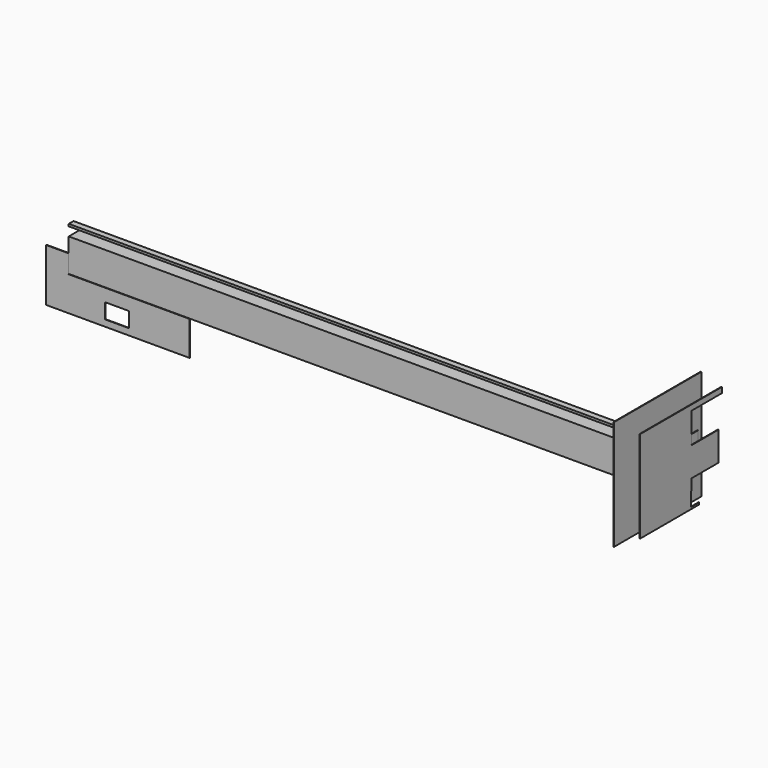
from build123d import *

# Parameters (mm, degrees)
F0_W      = 1666.3101315498
F0_H      = 1440.3567910194
F0_W_2    = 321.9513893127
F0_H_2    = 173.8705039024
F1_DEPTH  = 25.4
F2_W      = 601.3025641441
F2_H      = 270.2689170837
F2_W_2    = 546.2159514427
F2_H_2    = 393.4317827225
F2_W_3    = 484.9420785904
F2_H_3    = 512.361317873
F2_W_4    = 315.6808614731
F2_H_4    = 497.0915317535
F2_W_5    = 263.4772062302
F2_H_5    = 414.9414896965
F3_DEPTH  = 25.4
F4_W      = 1832.0484161377
F4_H      = 3807.0937395096
F5_DEPTH  = 25.4
F6_W      = 670.0121164322
F6_H      = 1531.9002270699
F6_W_2    = 276.8320441246
F6_H_2    = 106.2819361687
F7_DEPTH  = 28066.4691925049
F8_W      = 5071.1117982864
F8_H      = 5097.4462032318
F9_DEPTH  = 25.4
F10_W     = 1443.1173034668
F10_H     = 1491.5601015091
F10_W_2   = 1109.7354888916
F10_H_2   = 703.5193443298
F10_W_3   = 2133.3904266357
F10_H_3   = 1594.1830873489
F11_DEPTH = 25.4
F12_W     = 2353.1031608582
F12_H     = 645.3219652176
F12_H_2   = 89.3001556396
F12_W_2   = 1552.1093606949
F12_H_3   = 1351.4214754105
F12_W_3   = 466.8933153152
F13_DEPTH = 25.4


with BuildPart() as f1:
    # F0 (on Right) → F1 (new body)
    with BuildSketch(Plane.YZ):
        with Locations((-82.8691422939, -112.1042668819)):
            Rectangle(F0_W, F0_H)
        with Locations((160.9756946564, 86.9352519512)):
            Rectangle(F0_W_2, F0_H_2, mode=Mode.SUBTRACT)
    extrude(amount=F1_DEPTH)

    # F2 (on face) → F3 (join)
    with BuildSketch(Plane.YZ.offset(25.4)):
        Polygon((601.3025641441, -1092.7692651749), (901.9212722778, -1092.7692651749), (901.9212722778, -524.1619944572), (901.9212722778, 428.5740554333), (901.9212722778, 856.0312390327), (-642.5161361694, 856.0312390327), (-1059.429526329, 856.0312390327), (-1059.429526329, 658.6785316467), (-1059.429526329, 243.7370419502), (-1059.429526329, -191.7653083801), (-1059.429526329, -688.8568401337), (-1059.429526329, -1092.7692651749), (-1031.0319662094, -1092.7692651749), (-484.8160147667, -1092.7692651749), (0, -1092.7692651749), align=None)
        with Locations((300.6512820721, -1227.9037237167)):
            Rectangle(F2_W, F2_H)
        Polygon((901.9212722778, 428.5740554333), (901.9212722778, -524.1619944572), (1412.9276275635, -524.1619944572), (1412.9276275635, 428.5740554333), (927.9855489731, 428.5740554333), align=None)
        Polygon((901.9212722778, 856.0312390327), (901.9212722778, 428.5740554333), (927.9855489731, 428.5740554333), (927.9855489731, 940.9353733063), (-642.5161361694, 940.9353733063), (-642.5161361694, 856.0312390327), align=None)
        with Locations((-757.9239904881, -1289.4851565361)):
            Rectangle(F2_W_2, F2_H_2)
        with Locations((1170.4565882683, 684.7547143698)):
            Rectangle(F2_W_3, F2_H_3)
        Polygon((-1059.429526329, 856.0312390327), (-642.5161361694, 856.0312390327), (-642.5161361694, 940.9353733063), (-642.5161361694, 1006.4268112183), (-1059.429526329, 1006.4268112183), align=None)
        Polygon((-642.5161361694, 940.9353733063), (927.9855489731, 940.9353733063), (927.9855489731, 1309.6973896027), (-642.5161361694, 1309.6973896027), (-642.5161361694, 1006.4268112183), align=None)
        with Locations((-1217.2699570656, -440.3110742569)):
            Rectangle(F2_W_4, F2_H_4)
        with Locations((-1191.1681294441, 451.2077867985)):
            Rectangle(F2_W_5, F2_H_5)
    extrude(amount=F3_DEPTH)

    # F4 (on face) → F5 (join)
    with BuildSketch(Plane(origin=(0, 0, 0), x_dir=(0, -1, 0), z_dir=(-1, 0, 0))):
        with Locations((916.0242080688, 681.5358996391)):
            Rectangle(F4_W, F4_H)
    extrude(amount=F5_DEPTH)

    # F6 (on face) → F7 (join)
    with BuildSketch(Plane(origin=(25.4, 0, 0), x_dir=(0, -1, 0), z_dir=(-1, 0, 0))):
        with Locations((-335.0060582161, -461.9536101818)):
            Rectangle(F6_W, F6_H)
        with Locations((-138.4160220623, 766.5357291698)):
            Rectangle(F6_W_2, F6_H_2)
    extrude(amount=F7_DEPTH)

    # F8 (on face) → F9 (join)
    with BuildSketch(Plane.YZ):
        with Locations((-907.9238772392, 686.8742704391)):
            Rectangle(F8_W, F8_H)
    extrude(amount=F9_DEPTH)

    # F12 (on face) → F13 (join)
    with BuildSketch(Plane.YZ.offset(50.8)):
        Polygon((-1996.6151714325, 2172.7378368378), (-1996.6151714325, 1918.0111885071), (-1375.1103878021, 1918.0111885071), (1005.3068399429, 1918.0111885071), (2760.6105804443, 1918.0111885071), (2760.6105804443, 2172.7378368378), align=None)
        Polygon((-1375.1103878021, 1918.0111885071), (-1996.6151714325, 1918.0111885071), (-1996.6151714325, -2097.6603031158), (-1375.1103878021, -2097.6603031158), (-1375.1103878021, -2008.3601474762), (-1375.1103878021, -1363.0381822586), align=None)
        Polygon((1005.3068399429, 1918.0111885071), (-1375.1103878021, 1918.0111885071), (-1375.1103878021, -1363.0381822586), (977.992773056, -1363.0381822586), (1005.3068399429, -1363.0381822586), (1005.3068399429, -843.8047766685), (1005.3068399429, 507.6166987419), align=None)
        with Locations((-198.558807373, -1685.6991648674)):
            Rectangle(F12_W, F12_H)
        with Locations((-198.558807373, -2053.010225296)):
            Rectangle(F12_W, F12_H_2)
        with Locations((1781.3615202904, -168.0940389633)):
            Rectangle(F12_W_2, F12_H_3)
        with Locations((1211.4394307137, -2053.010225296)):
            Rectangle(F12_W_3, F12_H_2)
    extrude(amount=F13_DEPTH)


with BuildPart() as f11:
    # F10 (on face) → F11 (new body)
    with BuildSketch(Plane.XZ):
        with Locations((-27319.5105407715, -1973.6837744713)):
            Rectangle(F10_W, F10_H)
        Polygon((-28041.0691925049, -2719.4638252258), (-28041.0691925049, -1227.9037237167), (-28041.0691925049, -372.6229667664), (-29072.9331970215, -372.6229667664), (-29072.9331970215, -2822.0868110657), (-28041.0691925049, -2822.0868110657), align=None)
        Polygon((-24540.3938293457, -1227.9037237167), (-26597.9518890381, -1227.9037237167), (-26597.9518890381, -2719.4638252258), (-28041.0691925049, -2719.4638252258), (-28041.0691925049, -2822.0868110657), (-24540.3938293457, -2822.0868110657), align=None)
        with Locations((-25781.0010910034, -2170.9516048431)):
            Rectangle(F10_W_2, F10_H_2, mode=Mode.SUBTRACT)
        with Locations((-23473.6986160278, -2024.9952673912)):
            Rectangle(F10_W_3, F10_H_3)
    extrude(amount=F11_DEPTH)


solid = Compound([f1.part, f11.part])
